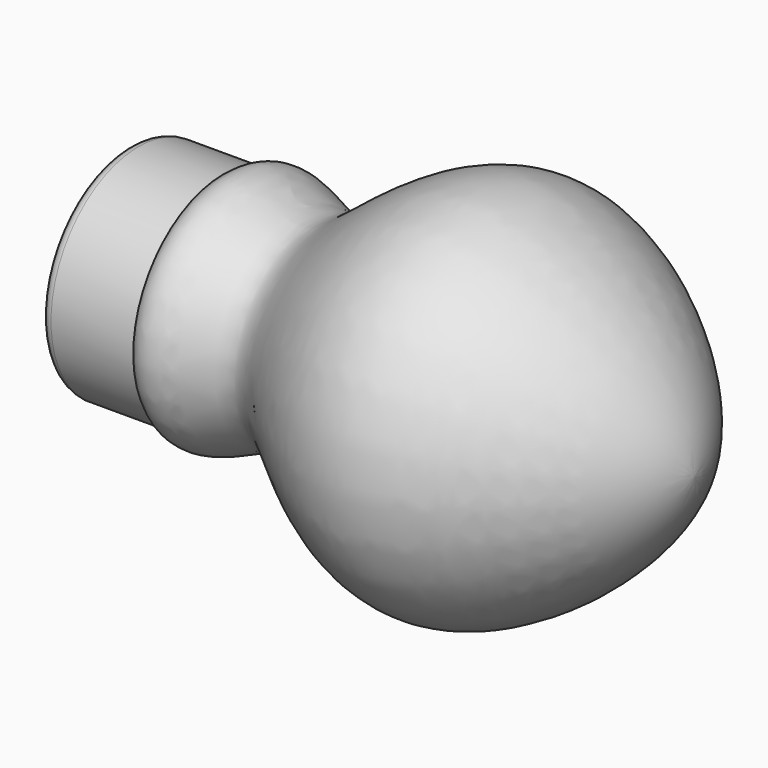
from build123d import *

# Parameters (mm, degrees)
F3_R     = 10.3
F3_R_2   = 9.3
F4_DEPTH = 7.9747296804
F3_R_3   = 4
F5_DEPTH = 1
F6_R     = 0.99999


# Not quite as in the source:
# - a fillet or chamfer is up to 0.001 mm smaller than in the source, because OpenCascade refuses the exact size


with BuildPart() as f1:
    # F0 (on Front) → F1 (revolve)
    with BuildSketch(Plane.XZ):
        with BuildLine():
            Line((-34.4216992354, 13.8474768028), (-42.4016992354, 13.8474768028))
            Line((-42.4016992354, 13.8474768028), (-42.3964289158, 8.5474768028))
            Line((-42.3964289158, 8.5474768028), (-19.3924513161, 8.5474768028))
            Line((-19.3924513161, 8.5474768028), (-19.3924513161, 4.5474768028))
            Line((-19.3924513161, 4.5474768028), (-16.721310094, 4.5474768028))
            Line((-16.721310094, 4.5474768028), (9.9075486839, 4.5474768028))
            add(Edge.make_bspline(
                [(-34.4216992354, 15.1406228542), (-32.625882799, 16.7578682962), (-27.4007330199, 13.1812527445), (-23.3492915473, 14.5315919009), (-8.9306439772, 29.2285299601), (9.6598378671, 10.9895048612), (9.9075486839, 4.5474768028)],
                knots=[0, 0, 0, 0, 0.1898510794, 0.3368036599, 0.6314655551, 1, 1, 1, 1], degree=3))
            Line((-34.4216992354, 15.1406228542), (-34.4216992354, 13.8474768028))
        make_face()
    revolve(axis=Axis((-3.4068807051, 0, 4.5474768028), (1, 0, 0)))


with BuildPart() as f4:
    # F3 (on plane+point) → F4 (new body, through all)
    with BuildSketch(Plane.YZ.offset(-42.3964289158)):
        with Locations((0, 4.5474768028)):
            Circle(F3_R)
        with Locations((0, 4.5474768028)):
            Circle(F3_R_2, mode=Mode.SUBTRACT)
    extrude(amount=F4_DEPTH)

    # F3 (on plane+point) → F5 (join)
    with BuildSketch(Plane.YZ.offset(-42.3964289158)):
        with Locations((0, 4.5474768028)):
            Circle(F3_R)
        with Locations((0, 4.5474768028)):
            Circle(F3_R_2, mode=Mode.SUBTRACT)
        with Locations((0, 4.5474768028)):
            Circle(F3_R_2)
        with Locations((0, 4.5474768028)):
            Circle(F3_R_3, mode=Mode.SUBTRACT)
    extrude(amount=-F5_DEPTH)

    # F6 (radius 1 in the source; OpenCascade refuses exactly that, so slightly less here)
    f6_edges = [f4.edges().sort_by_distance(p)[0] for p in [
        (-43.396429, -10.3, 4.547477),
    ]]
    fillet(f6_edges, radius=F6_R)


solid = Compound([f1.part, f4.part])
